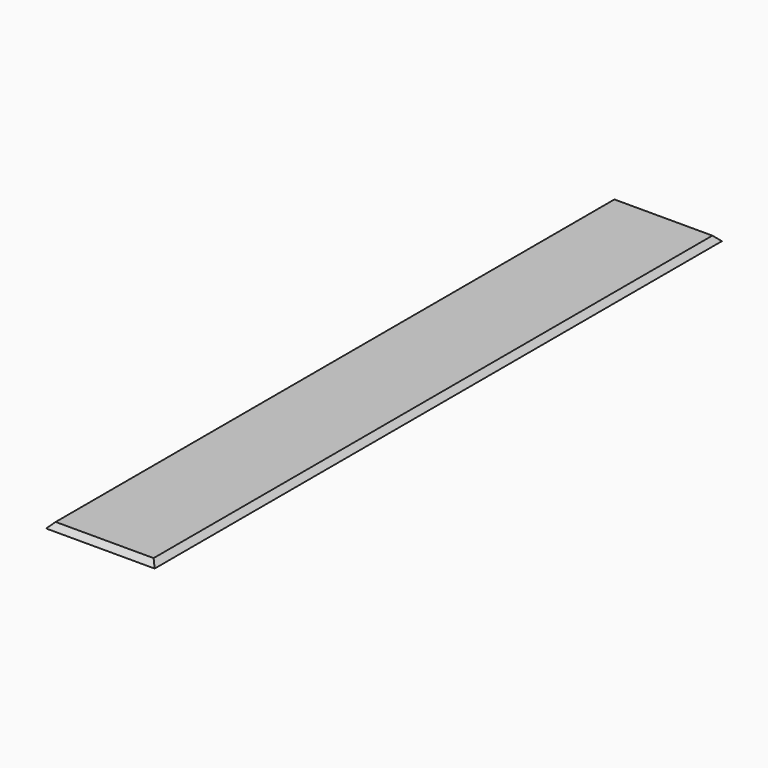
from build123d import *

# Parameters (mm, degrees)
F0_W     = 245
F0_H     = 1600
F1_DEPTH = 12
F2_SIZE  = 11.99999


# Not quite as in the source:
# - a fillet or chamfer is up to 0.001 mm smaller than in the source, because OpenCascade refuses the exact size


with BuildPart() as f1:
    # F0 (on Top) → F1 (new body)
    with BuildSketch(Plane.XY):
        Rectangle(F0_W, F0_H)
    extrude(amount=-F1_DEPTH)

    # F2 (size 12 in the source; OpenCascade refuses exactly that, so slightly less here)
    f2_edges = [f1.edges().sort_by_distance(p)[0] for p in [
        (0, -800, 0),
        (122.5, 0, 0),
        (-122.5, 0, 0),
        (0, 800, 0),
    ]]
    chamfer(f2_edges, length=F2_SIZE)


solid = f1.part
